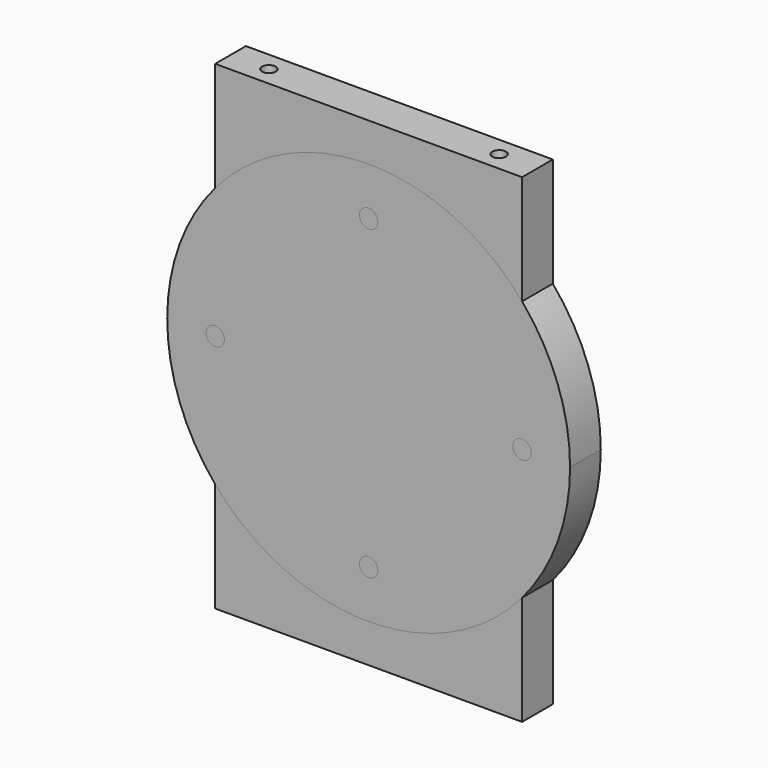
from build123d import *

# Parameters (mm, degrees)
F2_R      = 4.7625
F2_R_2    = 17.4625
F2_R_3    = 3.175
F5_DEPTH  = 6.35
F6_DEPTH  = 3.175
F7_D      = 3.048
F8_D      = 2.2606
F8_DEPTH  = 12.7
F8_TIP    = 0.6791527577
F9_D      = 2.2606
F9_DEPTH  = 12.7
F9_TIP    = 0.6791527577
F2_R_4    = 1
F2_R_5    = 8
F10_DEPTH = 6.35
F11_DEPTH = 3.175
F12_D     = 3.048
F13_DEPTH = 6.35
F14_DEPTH = 3.175
F15_D     = 3.048
F16_D     = 2.2606
F16_DEPTH = 12.7
F16_TIP   = 0.6791527577
F17_D     = 2.2606
F17_DEPTH = 12.7
F17_TIP   = 0.6791527577
F18_DEPTH = 6.35
F19_DEPTH = 3.175
F20_D     = 3.048


with BuildPart() as f5:
    # F2 (on Front) → F5 (new body)
    with BuildSketch(Plane.XZ):
        with BuildLine():
            ThreePointArc((25.4, -21.5923344326), (31.2902653093, -11.5025302923), (33.3375, 0))
            ThreePointArc((33.3375, 0), (31.2902653093, 11.5025302923), (25.4, 21.5923344326))
            ThreePointArc((25.4, 21.5923344326), (0, 33.3375), (-25.4, 21.5923344326))
            ThreePointArc((-25.4, 21.5923344326), (-33.3375, 0), (-25.4, -21.5923344326))
            ThreePointArc((-25.4, -21.5923344326), (0, -33.3375), (25.4, -21.5923344326))
        make_face()
        with Locations((-17.9605122421, -17.9605122421)):
            Circle(F2_R, mode=Mode.SUBTRACT)
        with Locations((0, -25.4)):
            Circle(F2_R, mode=Mode.SUBTRACT)
        with Locations((17.9605122421, -17.9605122421)):
            Circle(F2_R, mode=Mode.SUBTRACT)
        with Locations((-25.4, 0)):
            Circle(F2_R, mode=Mode.SUBTRACT)
        with Locations((-17.9605122421, 17.9605122421)):
            Circle(F2_R, mode=Mode.SUBTRACT)
        Circle(F2_R_2, mode=Mode.SUBTRACT)
        with Locations((25.4, 0)):
            Circle(F2_R, mode=Mode.SUBTRACT)
        with Locations((17.9605122421, 17.9605122421)):
            Circle(F2_R, mode=Mode.SUBTRACT)
        with Locations((0, 25.4)):
            Circle(F2_R, mode=Mode.SUBTRACT)
        with BuildLine():
            Line((25.4, -39.6875), (25.4, -21.5923344326))
            ThreePointArc((25.4, -21.5923344326), (0, -33.3375), (-25.4, -21.5923344326))
            Line((-25.4, -21.5923344326), (-25.4, -39.6875))
            Line((-25.4, -39.6875), (25.4, -39.6875))
        make_face()
        with BuildLine():
            ThreePointArc((-25.4, 21.5923344326), (0, 33.3375), (25.4, 21.5923344326))
            Line((25.4, 21.5923344326), (25.4, 39.6875))
            Line((25.4, 39.6875), (-25.4, 39.6875))
            Line((-25.4, 39.6875), (-25.4, 21.5923344326))
        make_face()
        with Locations((0, -25.4)):
            Circle(F2_R)
        with Locations((0, -25.4)):
            Circle(F2_R_3, mode=Mode.SUBTRACT)
        with Locations((-25.4, 0)):
            Circle(F2_R)
        with Locations((-25.4, 0)):
            Circle(F2_R_3, mode=Mode.SUBTRACT)
        with Locations((17.9605122421, -17.9605122421)):
            Circle(F2_R)
        with Locations((17.9605122421, -17.9605122421)):
            Circle(F2_R_3, mode=Mode.SUBTRACT)
        with Locations((25.4, 0)):
            Circle(F2_R)
        with Locations((25.4, 0)):
            Circle(F2_R_3, mode=Mode.SUBTRACT)
        with Locations((17.9605122421, 17.9605122421)):
            Circle(F2_R)
        with Locations((17.9605122421, 17.9605122421)):
            Circle(F2_R_3, mode=Mode.SUBTRACT)
        with Locations((0, 25.4)):
            Circle(F2_R)
        with Locations((0, 25.4)):
            Circle(F2_R_3, mode=Mode.SUBTRACT)
        with Locations((-17.9605122421, 17.9605122421)):
            Circle(F2_R)
        with Locations((-17.9605122421, 17.9605122421)):
            Circle(F2_R_3, mode=Mode.SUBTRACT)
        with Locations((-17.9605122421, -17.9605122421)):
            Circle(F2_R)
        with Locations((-17.9605122421, -17.9605122421)):
            Circle(F2_R_3, mode=Mode.SUBTRACT)
        with Locations((0, -25.4)):
            Circle(F2_R_3)
        with Locations((17.9605122421, -17.9605122421)):
            Circle(F2_R_3)
        with Locations((25.4, 0)):
            Circle(F2_R_3)
        with Locations((-25.4, 0)):
            Circle(F2_R_3)
        with Locations((-17.9605122421, 17.9605122421)):
            Circle(F2_R_3)
        with Locations((-17.9605122421, -17.9605122421)):
            Circle(F2_R_3)
        with Locations((0, 25.4)):
            Circle(F2_R_3)
        with Locations((17.9605122421, 17.9605122421)):
            Circle(F2_R_3)
    extrude(amount=F5_DEPTH)

    # F2 (on Front) → F6 (cut)
    with BuildSketch(Plane.XZ):
        with Locations((17.9605122421, -17.9605122421)):
            Circle(F2_R_3)
        with Locations((17.9605122421, 17.9605122421)):
            Circle(F2_R_3)
        with Locations((-17.9605122421, 17.9605122421)):
            Circle(F2_R_3)
        with Locations((-17.9605122421, -17.9605122421)):
            Circle(F2_R_3)
    extrude(amount=F6_DEPTH, mode=Mode.SUBTRACT)

    # F7 (through all)
    with Locations(Plane(origin=(0, 0, 0), x_dir=(1, 0, 0), z_dir=(0, 1, 0))):
        with Locations((17.9605122421, -17.9605122421), (-17.9605122421, -17.9605122421), (-17.9605122421, 17.9605122421), (17.9605122421, 17.9605122421)):
            Hole(F7_D / 2)

    # F8
    with Locations(Plane.XY.offset(39.6875)):
        with Locations((-19.05, -3.175), (19.05, -3.175)):
            Hole(F8_D / 2, depth=F8_DEPTH)
            with Locations((0, 0, -(F8_DEPTH + F8_TIP / 2))):  # 118° drill point
                Cone(0, F8_D / 2, F8_TIP, mode=Mode.SUBTRACT)

    # F9
    with Locations(Plane(origin=(0, 0, -39.6875), x_dir=(1, 0, 0), z_dir=(0, 0, -1))):
        with Locations((-19.05, 3.175), (19.05, 3.175)):
            Hole(F9_D / 2, depth=F9_DEPTH)
            with Locations((0, 0, -(F9_DEPTH + F9_TIP / 2))):  # 118° drill point
                Cone(0, F9_D / 2, F9_TIP, mode=Mode.SUBTRACT)


with BuildPart() as f10:
    # F2 (on Front) → F10 (new body)
    with BuildSketch(Plane.XZ):
        with BuildLine():
            ThreePointArc((25.4, -21.5923344326), (31.2902653093, -11.5025302923), (33.3375, 0))
            ThreePointArc((33.3375, 0), (31.2902653093, 11.5025302923), (25.4, 21.5923344326))
            ThreePointArc((25.4, 21.5923344326), (0, 33.3375), (-25.4, 21.5923344326))
            ThreePointArc((-25.4, 21.5923344326), (-33.3375, 0), (-25.4, -21.5923344326))
            ThreePointArc((-25.4, -21.5923344326), (0, -33.3375), (25.4, -21.5923344326))
        make_face()
        with Locations((-17.9605122421, -17.9605122421)):
            Circle(F2_R, mode=Mode.SUBTRACT)
        with Locations((0, -25.4)):
            Circle(F2_R, mode=Mode.SUBTRACT)
        with Locations((17.9605122421, -17.9605122421)):
            Circle(F2_R, mode=Mode.SUBTRACT)
        with Locations((-25.4, 0)):
            Circle(F2_R, mode=Mode.SUBTRACT)
        with Locations((-17.9605122421, 17.9605122421)):
            Circle(F2_R, mode=Mode.SUBTRACT)
        Circle(F2_R_2, mode=Mode.SUBTRACT)
        with Locations((25.4, 0)):
            Circle(F2_R, mode=Mode.SUBTRACT)
        with Locations((17.9605122421, 17.9605122421)):
            Circle(F2_R, mode=Mode.SUBTRACT)
        with Locations((0, 25.4)):
            Circle(F2_R, mode=Mode.SUBTRACT)
        Circle(F2_R_2)
        with Locations((-8, -8)):
            Circle(F2_R_4, mode=Mode.SUBTRACT)
        with Locations((8, -8)):
            Circle(F2_R_4, mode=Mode.SUBTRACT)
        with Locations((-8, 8)):
            Circle(F2_R_4, mode=Mode.SUBTRACT)
        Circle(F2_R_5, mode=Mode.SUBTRACT)
        with Locations((8, 8)):
            Circle(F2_R_4, mode=Mode.SUBTRACT)
        with Locations((-25.4, 0)):
            Circle(F2_R)
        with Locations((-25.4, 0)):
            Circle(F2_R_3, mode=Mode.SUBTRACT)
        with Locations((0, -25.4)):
            Circle(F2_R)
        with Locations((0, -25.4)):
            Circle(F2_R_3, mode=Mode.SUBTRACT)
        with Locations((25.4, 0)):
            Circle(F2_R)
        with Locations((25.4, 0)):
            Circle(F2_R_3, mode=Mode.SUBTRACT)
        with Locations((0, 25.4)):
            Circle(F2_R)
        with Locations((0, 25.4)):
            Circle(F2_R_3, mode=Mode.SUBTRACT)
        with Locations((-25.4, 0)):
            Circle(F2_R_3)
        with Locations((0, -25.4)):
            Circle(F2_R_3)
        with Locations((25.4, 0)):
            Circle(F2_R_3)
        with Locations((0, 25.4)):
            Circle(F2_R_3)
    extrude(amount=F10_DEPTH)

    # F2 (on Front) → F11 (cut)
    with BuildSketch(Plane.XZ):
        with Locations((0, 25.4)):
            Circle(F2_R_3)
        with Locations((-25.4, 0)):
            Circle(F2_R_3)
        with Locations((0, -25.4)):
            Circle(F2_R_3)
        with Locations((25.4, 0)):
            Circle(F2_R_3)
    extrude(amount=F11_DEPTH, mode=Mode.SUBTRACT)

    # F12 (through all)
    with Locations(Plane(origin=(0, 0, 0), x_dir=(1, 0, 0), z_dir=(0, 1, 0))):
        with Locations((25.4, 0), (0, -25.4), (-25.4, 0), (0, 25.4)):
            Hole(F12_D / 2)


with BuildPart() as f13:
    # F2 (on Front) → F13 (new body)
    with BuildSketch(Plane.XZ):
        with BuildLine():
            ThreePointArc((25.4, -21.5923344326), (31.2902653093, -11.5025302923), (33.3375, 0))
            ThreePointArc((33.3375, 0), (31.2902653093, 11.5025302923), (25.4, 21.5923344326))
            ThreePointArc((25.4, 21.5923344326), (0, 33.3375), (-25.4, 21.5923344326))
            ThreePointArc((-25.4, 21.5923344326), (-33.3375, 0), (-25.4, -21.5923344326))
            ThreePointArc((-25.4, -21.5923344326), (0, -33.3375), (25.4, -21.5923344326))
        make_face()
        with Locations((-17.9605122421, -17.9605122421)):
            Circle(F2_R, mode=Mode.SUBTRACT)
        with Locations((0, -25.4)):
            Circle(F2_R, mode=Mode.SUBTRACT)
        with Locations((17.9605122421, -17.9605122421)):
            Circle(F2_R, mode=Mode.SUBTRACT)
        with Locations((-25.4, 0)):
            Circle(F2_R, mode=Mode.SUBTRACT)
        with Locations((-17.9605122421, 17.9605122421)):
            Circle(F2_R, mode=Mode.SUBTRACT)
        Circle(F2_R_2, mode=Mode.SUBTRACT)
        with Locations((25.4, 0)):
            Circle(F2_R, mode=Mode.SUBTRACT)
        with Locations((17.9605122421, 17.9605122421)):
            Circle(F2_R, mode=Mode.SUBTRACT)
        with Locations((0, 25.4)):
            Circle(F2_R, mode=Mode.SUBTRACT)
        Circle(F2_R_2)
        with Locations((-8, -8)):
            Circle(F2_R_4, mode=Mode.SUBTRACT)
        with Locations((8, -8)):
            Circle(F2_R_4, mode=Mode.SUBTRACT)
        with Locations((-8, 8)):
            Circle(F2_R_4, mode=Mode.SUBTRACT)
        Circle(F2_R_5, mode=Mode.SUBTRACT)
        with Locations((8, 8)):
            Circle(F2_R_4, mode=Mode.SUBTRACT)
        with BuildLine():
            ThreePointArc((-25.4, 21.5923344326), (0, 33.3375), (25.4, 21.5923344326))
            Line((25.4, 21.5923344326), (25.4, 39.6875))
            Line((25.4, 39.6875), (-25.4, 39.6875))
            Line((-25.4, 39.6875), (-25.4, 21.5923344326))
        make_face()
        with BuildLine():
            Line((25.4, -39.6875), (25.4, -21.5923344326))
            ThreePointArc((25.4, -21.5923344326), (0, -33.3375), (-25.4, -21.5923344326))
            Line((-25.4, -21.5923344326), (-25.4, -39.6875))
            Line((-25.4, -39.6875), (25.4, -39.6875))
        make_face()
        Circle(F2_R_5)
        Polygon((0, 7.3323484187), (6.35, 3.6661742094), (6.35, -3.6661742094), (0, -7.3323484187), (-6.35, -3.6661742094), (-6.35, 3.6661742094), align=None, mode=Mode.SUBTRACT)
        with Locations((17.9605122421, 17.9605122421)):
            Circle(F2_R)
        with Locations((17.9605122421, 17.9605122421)):
            Circle(F2_R_3, mode=Mode.SUBTRACT)
        with Locations((17.9605122421, -17.9605122421)):
            Circle(F2_R)
        with Locations((17.9605122421, -17.9605122421)):
            Circle(F2_R_3, mode=Mode.SUBTRACT)
        with Locations((-17.9605122421, -17.9605122421)):
            Circle(F2_R)
        with Locations((-17.9605122421, -17.9605122421)):
            Circle(F2_R_3, mode=Mode.SUBTRACT)
        with Locations((-17.9605122421, 17.9605122421)):
            Circle(F2_R)
        with Locations((-17.9605122421, 17.9605122421)):
            Circle(F2_R_3, mode=Mode.SUBTRACT)
        with Locations((17.9605122421, 17.9605122421)):
            Circle(F2_R_3)
        with Locations((17.9605122421, -17.9605122421)):
            Circle(F2_R_3)
        with Locations((-17.9605122421, 17.9605122421)):
            Circle(F2_R_3)
        with Locations((-17.9605122421, -17.9605122421)):
            Circle(F2_R_3)
        with Locations((8, -8)):
            Circle(F2_R_4)
        with Locations((-8, 8)):
            Circle(F2_R_4)
        with Locations((8, 8)):
            Circle(F2_R_4)
        with Locations((-8, -8)):
            Circle(F2_R_4)
    extrude(amount=F13_DEPTH)

    # F2 (on Front) → F14 (cut)
    with BuildSketch(Plane.XZ):
        with Locations((17.9605122421, -17.9605122421)):
            Circle(F2_R_3)
        with Locations((17.9605122421, 17.9605122421)):
            Circle(F2_R_3)
        with Locations((-17.9605122421, 17.9605122421)):
            Circle(F2_R_3)
        with Locations((-17.9605122421, -17.9605122421)):
            Circle(F2_R_3)
    extrude(amount=F14_DEPTH, mode=Mode.SUBTRACT)

    # F15 (through all)
    with Locations(Plane(origin=(0, 0, 0), x_dir=(1, 0, 0), z_dir=(0, 1, 0))):
        with Locations((17.9605122421, -17.9605122421), (-17.9605122421, -17.9605122421), (-17.9605122421, 17.9605122421), (17.9605122421, 17.9605122421)):
            Hole(F15_D / 2)

    # F16
    with Locations(Plane.XY.offset(39.6875)):
        with Locations((-19.05, -3.175), (19.05, -3.175)):
            Hole(F16_D / 2, depth=F16_DEPTH)
            with Locations((0, 0, -(F16_DEPTH + F16_TIP / 2))):  # 118° drill point
                Cone(0, F16_D / 2, F16_TIP, mode=Mode.SUBTRACT)

    # F17
    with Locations(Plane(origin=(0, 0, -39.6875), x_dir=(1, 0, 0), z_dir=(0, 0, -1))):
        with Locations((-19.05, 3.175), (19.05, 3.175)):
            Hole(F17_D / 2, depth=F17_DEPTH)
            with Locations((0, 0, -(F17_DEPTH + F17_TIP / 2))):  # 118° drill point
                Cone(0, F17_D / 2, F17_TIP, mode=Mode.SUBTRACT)


with BuildPart() as f18:
    # F2 (on Front) → F18 (new body)
    with BuildSketch(Plane.XZ):
        with BuildLine():
            ThreePointArc((25.4, -21.5923344326), (31.2902653093, -11.5025302923), (33.3375, 0))
            ThreePointArc((33.3375, 0), (31.2902653093, 11.5025302923), (25.4, 21.5923344326))
            ThreePointArc((25.4, 21.5923344326), (0, 33.3375), (-25.4, 21.5923344326))
            ThreePointArc((-25.4, 21.5923344326), (-33.3375, 0), (-25.4, -21.5923344326))
            ThreePointArc((-25.4, -21.5923344326), (0, -33.3375), (25.4, -21.5923344326))
        make_face()
        with Locations((-17.9605122421, -17.9605122421)):
            Circle(F2_R, mode=Mode.SUBTRACT)
        with Locations((0, -25.4)):
            Circle(F2_R, mode=Mode.SUBTRACT)
        with Locations((17.9605122421, -17.9605122421)):
            Circle(F2_R, mode=Mode.SUBTRACT)
        with Locations((-25.4, 0)):
            Circle(F2_R, mode=Mode.SUBTRACT)
        with Locations((-17.9605122421, 17.9605122421)):
            Circle(F2_R, mode=Mode.SUBTRACT)
        Circle(F2_R_2, mode=Mode.SUBTRACT)
        with Locations((25.4, 0)):
            Circle(F2_R, mode=Mode.SUBTRACT)
        with Locations((17.9605122421, 17.9605122421)):
            Circle(F2_R, mode=Mode.SUBTRACT)
        with Locations((0, 25.4)):
            Circle(F2_R, mode=Mode.SUBTRACT)
        Circle(F2_R_2)
        with Locations((-8, -8)):
            Circle(F2_R_4, mode=Mode.SUBTRACT)
        with Locations((8, -8)):
            Circle(F2_R_4, mode=Mode.SUBTRACT)
        with Locations((-8, 8)):
            Circle(F2_R_4, mode=Mode.SUBTRACT)
        Circle(F2_R_5, mode=Mode.SUBTRACT)
        with Locations((8, 8)):
            Circle(F2_R_4, mode=Mode.SUBTRACT)
        Circle(F2_R_5)
        Polygon((0, 7.3323484187), (6.35, 3.6661742094), (6.35, -3.6661742094), (0, -7.3323484187), (-6.35, -3.6661742094), (-6.35, 3.6661742094), align=None, mode=Mode.SUBTRACT)
        Polygon((6.35, -3.6661742094), (6.35, 3.6661742094), (0, 7.3323484187), (-6.35, 3.6661742094), (-6.35, -3.6661742094), (0, -7.3323484187), align=None)
        with Locations((0, -25.4)):
            Circle(F2_R)
        with Locations((0, -25.4)):
            Circle(F2_R_3, mode=Mode.SUBTRACT)
        with Locations((0, 25.4)):
            Circle(F2_R)
        with Locations((0, 25.4)):
            Circle(F2_R_3, mode=Mode.SUBTRACT)
        with Locations((-25.4, 0)):
            Circle(F2_R)
        with Locations((-25.4, 0)):
            Circle(F2_R_3, mode=Mode.SUBTRACT)
        with Locations((17.9605122421, 17.9605122421)):
            Circle(F2_R)
        with Locations((17.9605122421, 17.9605122421)):
            Circle(F2_R_3, mode=Mode.SUBTRACT)
        with Locations((25.4, 0)):
            Circle(F2_R)
        with Locations((25.4, 0)):
            Circle(F2_R_3, mode=Mode.SUBTRACT)
        with Locations((17.9605122421, -17.9605122421)):
            Circle(F2_R)
        with Locations((17.9605122421, -17.9605122421)):
            Circle(F2_R_3, mode=Mode.SUBTRACT)
        with Locations((-17.9605122421, -17.9605122421)):
            Circle(F2_R)
        with Locations((-17.9605122421, -17.9605122421)):
            Circle(F2_R_3, mode=Mode.SUBTRACT)
        with Locations((-17.9605122421, 17.9605122421)):
            Circle(F2_R)
        with Locations((-17.9605122421, 17.9605122421)):
            Circle(F2_R_3, mode=Mode.SUBTRACT)
        with Locations((25.4, 0)):
            Circle(F2_R_3)
        with Locations((17.9605122421, 17.9605122421)):
            Circle(F2_R_3)
        with Locations((17.9605122421, -17.9605122421)):
            Circle(F2_R_3)
        with Locations((-25.4, 0)):
            Circle(F2_R_3)
        with Locations((0, 25.4)):
            Circle(F2_R_3)
        with Locations((-17.9605122421, 17.9605122421)):
            Circle(F2_R_3)
        with Locations((-17.9605122421, -17.9605122421)):
            Circle(F2_R_3)
        with Locations((0, -25.4)):
            Circle(F2_R_3)
        with Locations((-8, 8)):
            Circle(F2_R_4)
        with Locations((-8, -8)):
            Circle(F2_R_4)
        with Locations((8, 8)):
            Circle(F2_R_4)
        with Locations((8, -8)):
            Circle(F2_R_4)
    extrude(amount=F18_DEPTH)

    # F2 (on Front) → F19 (cut)
    with BuildSketch(Plane.XZ):
        with Locations((0, 25.4)):
            Circle(F2_R_3)
        with Locations((25.4, 0)):
            Circle(F2_R_3)
        with Locations((0, -25.4)):
            Circle(F2_R_3)
        with Locations((-25.4, 0)):
            Circle(F2_R_3)
    extrude(amount=F19_DEPTH, mode=Mode.SUBTRACT)

    # F20 (through all)
    with Locations(Plane(origin=(0, 0, 0), x_dir=(1, 0, 0), z_dir=(0, 1, 0))):
        with Locations((25.4, 0), (0, -25.4), (-25.4, 0), (0, 25.4)):
            Hole(F20_D / 2)


solid = Compound([f5.part, f10.part, f13.part, f18.part])
